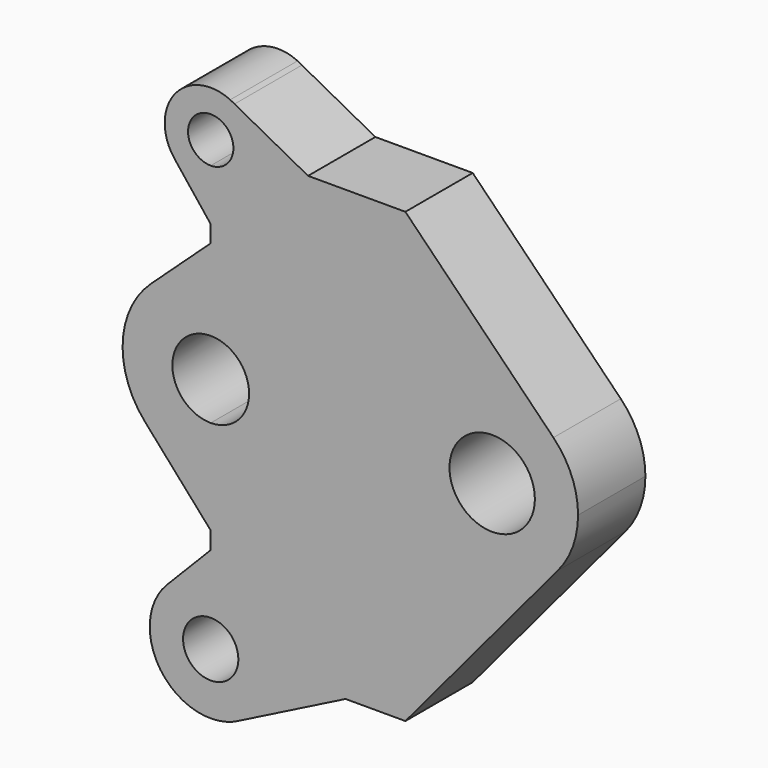
from build123d import *

# Parameters (mm, degrees)
F0_R     = 12.8832343864
F1_DEPTH = 25.4


with BuildPart() as f1:
    # F0 (on Front) → F1 (new body)
    with BuildSketch(Plane.XZ):
        with BuildLine():
            ThreePointArc((35.9714085189, -16.6367422783), (40.4577681305, -8.850339279), (42.0156477411, 0))
            ThreePointArc((42.0156477411, 0), (40.0854751838, 9.8147034219), (34.5824417765, 18.1675827265))
            ThreePointArc((34.5824417765, 18.1675827265), (-9.8005378371, -1.0335256515), (35.9714085189, -16.6367422783))
        make_face()
        with Locations((16.0972476006, 0)):
            Circle(F0_R, mode=Mode.SUBTRACT)
        with BuildLine():
            ThreePointArc((35.9714085189, -16.6367422783), (-9.8005378371, -1.0335256515), (34.5824417765, 18.1675827265))
            Line((34.5824417765, 18.1675827265), (-10.098147206, 63.6292919517))
            Line((-10.098147206, 63.6292919517), (-10.098147206, -71.6711804271))
            Line((-10.098147206, -71.6711804271), (35.9714085189, -16.6367422783))
        make_face()
        with BuildLine():
            Line((-10.098147206, -71.6711804271), (-10.098147206, 63.6292919517))
            Line((-10.098147206, 63.6292919517), (-39.4725925289, 63.6292919517))
            Line((-39.4725925289, 63.6292919517), (-54.9636371203, 63.6292919517))
            ThreePointArc((-54.9636371203, 63.6292919517), (-59.0299910486, 53.8122451485), (-68.8470378518, 49.7458912202))
            Line((-68.8470378518, 49.7458912202), (-68.8470378518, 41.2487648427))
            Line((-68.8470378518, 41.2487648427), (-68.8470378518, 36.1622795463))
            Line((-68.8470378518, 36.1622795463), (-68.8470378518, 26.5920495883))
            ThreePointArc((-68.8470378518, 26.5920495883), (-50.0436192623, 18.8034185895), (-42.2549882636, 0))
            ThreePointArc((-42.2549882636, 0), (-50.0436192623, -18.8034185895), (-68.8470378518, -26.5920495883))
            Line((-68.8470378518, -26.5920495883), (-68.8470378518, -40.1349775493))
            Line((-68.8470378518, -40.1349775493), (-68.8470378518, -45.3523172626))
            Line((-68.8470378518, -45.3523172626), (-68.8470378518, -53.2724790463))
            ThreePointArc((-68.8470378518, -53.2724790463), (-55.8371913405, -58.6613339157), (-50.4483364711, -71.6711804271))
            Line((-50.4483364711, -71.6711804271), (-28.1551647931, -71.6711804271))
            Line((-28.1551647931, -71.6711804271), (-10.098147206, -71.6711804271))
        make_face()
        with BuildLine():
            Line((-54.9636371203, 63.6292919517), (-39.4725925289, 63.6292919517))
            Line((-39.4725925289, 63.6292919517), (-61.649666293, 75.5013877445))
            ThreePointArc((-61.649666293, 75.5013877445), (-56.7500793614, 70.4419574471), (-54.9636371203, 63.6292919517))
        make_face()
        with BuildLine():
            Line((-59.4641008402, -87.49750993), (-28.1551647931, -71.6711804271))
            Line((-28.1551647931, -71.6711804271), (-50.4483364711, -71.6711804271))
            ThreePointArc((-50.4483364711, -71.6711804271), (-52.8603860972, -80.7782753631), (-59.4641008402, -87.49750993))
        make_face()
        with BuildLine():
            Line((-62.0038737832, 63.6292919517), (-54.9636371203, 63.6292919517))
            ThreePointArc((-54.9636371203, 63.6292919517), (-56.7500793614, 70.4419574471), (-61.649666293, 75.5013877445))
            Line((-61.649666293, 75.5013877445), (-62.9583441397, 76.2019647875))
            ThreePointArc((-62.9583441397, 76.2019647875), (-79.7306355491, 72.2488114878), (-79.7363139169, 55.0169471694))
            ThreePointArc((-79.7363139169, 55.0169471694), (-74.8960122286, 51.1329434906), (-68.8470378518, 49.7458912202))
            Line((-68.8470378518, 49.7458912202), (-68.8470378518, 56.786127883))
            ThreePointArc((-68.8470378518, 56.786127883), (-73.6858855695, 68.4681396694), (-62.0038737832, 63.6292919517))
        make_face()
        with BuildLine():
            ThreePointArc((-68.8470378518, 49.7458912202), (-59.0299910486, 53.8122451485), (-54.9636371203, 63.6292919517))
            Line((-54.9636371203, 63.6292919517), (-62.0038737832, 63.6292919517))
            ThreePointArc((-62.0038737832, 63.6292919517), (-64.0081901341, 58.790444234), (-68.8470378518, 56.786127883))
            Line((-68.8470378518, 56.786127883), (-68.8470378518, 49.7458912202))
        make_face()
        with BuildLine():
            Line((-60.5045882043, -71.6711804271), (-50.4483364711, -71.6711804271))
            ThreePointArc((-50.4483364711, -71.6711804271), (-55.8371913405, -58.6613339157), (-68.8470378518, -53.2724790463))
            Line((-68.8470378518, -53.2724790463), (-68.8470378518, -63.3287307796))
            ThreePointArc((-68.8470378518, -63.3287307796), (-62.9480351344, -65.7721777096), (-60.5045882043, -71.6711804271))
        make_face()
        with BuildLine():
            ThreePointArc((-59.4641008402, -87.49750993), (-52.8603860972, -80.7782753631), (-50.4483364711, -71.6711804271))
            Line((-50.4483364711, -71.6711804271), (-60.5045882043, -71.6711804271))
            ThreePointArc((-60.5045882043, -71.6711804271), (-74.7460405693, -77.5701831445), (-68.8470378518, -63.3287307796))
            Line((-68.8470378518, -63.3287307796), (-68.8470378518, -53.2724790463))
            ThreePointArc((-68.8470378518, -53.2724790463), (-75.9838725238, -54.7130613284), (-82.0031068427, -58.8092186325))
            ThreePointArc((-82.0031068427, -58.8092186325), (-84.044592452, -82.0416455406), (-61.6670109584, -88.6110572362))
            Line((-61.6670109584, -88.6110572362), (-59.4641008402, -87.49750993))
        make_face()
        with BuildLine():
            Line((-68.8470378518, 41.2487648427), (-68.8470378518, 49.7458912202))
            ThreePointArc((-68.8470378518, 49.7458912202), (-74.8960122286, 51.1329434906), (-79.7363139169, 55.0169471694))
            Line((-79.7363139169, 55.0169471694), (-68.8470378518, 41.2487648427))
        make_face()
        with BuildLine():
            ThreePointArc((-82.0031068427, -58.8092186325), (-75.9838725238, -54.7130613284), (-68.8470378518, -53.2724790463))
            Line((-68.8470378518, -53.2724790463), (-68.8470378518, -45.3523172626))
            Line((-68.8470378518, -45.3523172626), (-82.0031068427, -58.8092186325))
        make_face()
        with BuildLine():
            Line((-68.8470378518, 26.5920495883), (-68.8470378518, 36.1622795463))
            Line((-68.8470378518, 36.1622795463), (-86.8680444269, 19.5545499393))
            ThreePointArc((-86.8680444269, 19.5545499393), (-78.5202363829, 24.7702711225), (-68.8470378518, 26.5920495883))
        make_face()
        with BuildLine():
            Line((-88.7645898629, -17.6189733864), (-68.8470378518, -40.1349775493))
            Line((-68.8470378518, -40.1349775493), (-68.8470378518, -26.5920495883))
            ThreePointArc((-68.8470378518, -26.5920495883), (-79.7697776024, -24.2452233985), (-88.7645898629, -17.6189733864))
        make_face()
        with BuildLine():
            Line((-68.8470378518, 11.5769225395), (-68.8470378518, 26.5920495883))
            ThreePointArc((-68.8470378518, 26.5920495883), (-78.5202363829, 24.7702711225), (-86.8680444269, 19.5545499393))
            ThreePointArc((-86.8680444269, 19.5545499393), (-95.4045465077, 1.3549299966), (-88.7645898629, -17.6189733864))
            ThreePointArc((-88.7645898629, -17.6189733864), (-79.7697776024, -24.2452233985), (-68.8470378518, -26.5920495883))
            Line((-68.8470378518, -26.5920495883), (-68.8470378518, -11.5769225395))
            ThreePointArc((-68.8470378518, -11.5769225395), (-80.4239603913, 0), (-68.8470378518, 11.5769225395))
        make_face()
        with BuildLine():
            ThreePointArc((-42.2549882636, 0), (-50.0436192623, 18.8034185895), (-68.8470378518, 26.5920495883))
            Line((-68.8470378518, 26.5920495883), (-68.8470378518, 11.5769225395))
            ThreePointArc((-68.8470378518, 11.5769225395), (-60.6609174189, 8.1861204329), (-57.2701153124, 0))
            ThreePointArc((-57.2701153124, 0), (-60.6609174189, -8.1861204329), (-68.8470378518, -11.5769225395))
            Line((-68.8470378518, -11.5769225395), (-68.8470378518, -26.5920495883))
            ThreePointArc((-68.8470378518, -26.5920495883), (-50.0436192623, -18.8034185895), (-42.2549882636, 0))
        make_face()
    extrude(amount=-F1_DEPTH)


solid = f1.part
